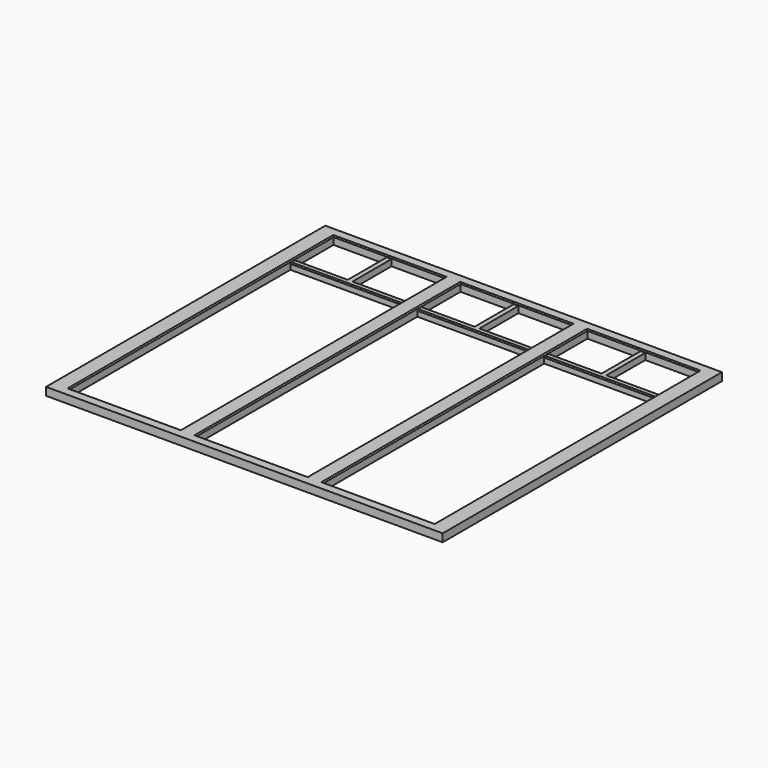
from build123d import *

# Parameters (mm, degrees)
F0_W      = 2500
F0_H      = 2200
F1_DEPTH  = 50
F0_W_2    = 30
F0_H_2    = 300
F2_DEPTH  = 40
F3_SIZE   = 7
F3_2_SIZE = 7
F3_3_SIZE = 7
F3_4_SIZE = 7


# Not quite as in the source:
# - a feature names something its author has since deleted; it is built from what else it names


with BuildPart() as f1:
    # F0 (on Top) → F1 (new body)
    with BuildSketch(Plane.XY):
        with Locations((321.0913794215, -344.7952681527)):
            Rectangle(F0_W, F0_H)
        Polygon((-828.9086205785, 395.2047318473), (-828.9086205785, 695.2047318473), (-493.9086205785, 695.2047318473), (-463.9086205785, 695.2047318473), (-128.9086205785, 695.2047318473), (-28.9086205785, 695.2047318473), (306.0913794215, 695.2047318473), (336.0913794215, 695.2047318473), (671.0913794215, 695.2047318473), (771.0913794215, 695.2047318473), (1106.0913794215, 695.2047318473), (1136.0913794215, 695.2047318473), (1471.0913794215, 695.2047318473), (1471.0913794215, 395.2047318473), (1471.0913794215, 355.2047318473), (1471.0913794215, -1384.7952681527), (771.0913794215, -1384.7952681527), (671.0913794215, -1384.7952681527), (-28.9086205785, -1384.7952681527), (-128.9086205785, -1384.7952681527), (-828.9086205785, -1384.7952681527), (-828.9086205785, 355.2047318473), align=None, mode=Mode.SUBTRACT)
        Polygon((-28.9086205785, 695.2047318473), (-128.9086205785, 695.2047318473), (-128.9086205785, 395.2047318473), (-128.9086205785, 355.2047318473), (-128.9086205785, -1384.7952681527), (-28.9086205785, -1384.7952681527), (-28.9086205785, 355.2047318473), (-28.9086205785, 395.2047318473), align=None)
        Polygon((671.0913794215, 355.2047318473), (671.0913794215, -1384.7952681527), (771.0913794215, -1384.7952681527), (771.0913794215, 355.2047318473), (771.0913794215, 395.2047318473), (771.0913794215, 695.2047318473), (671.0913794215, 695.2047318473), (671.0913794215, 395.2047318473), align=None)
    extrude(amount=F1_DEPTH)

    # F3
    f3_edges = [f1.edges().sort_by_distance(p)[0] for p in [
        (-828.908621, -344.795268, 50),
        (-478.908621, 695.204732, 50),
        (-128.908621, -344.795268, 50),
        (-28.908621, -344.795268, 50),
        (321.091379, 695.204732, 50),
        (771.091379, -344.795268, 50),
        (1121.091379, 695.204732, 50),
        (671.091379, -344.795268, 50),
        (1471.091379, -344.795268, 50),
        (321.091379, -1384.795268, 50),
        (1121.091379, -1384.795268, 50),
        (-478.908621, -1384.795268, 50),
    ]]
    chamfer(f3_edges, length=F3_SIZE)


with BuildPart() as f2:
    # F0 (on Top) → F2 (new body)
    with BuildSketch(Plane.XY):
        Polygon((-493.9086205785, 395.2047318473), (-828.9086205785, 395.2047318473), (-828.9086205785, 355.2047318473), (-128.9086205785, 355.2047318473), (-128.9086205785, 395.2047318473), (-463.9086205785, 395.2047318473), align=None)
        with Locations((-478.9086205785, 545.2047318473)):
            Rectangle(F0_W_2, F0_H_2)
    extrude(amount=F2_DEPTH)

    # F3#2
    f3_2_edges = [f2.edges().sort_by_distance(p)[0] for p in [
        (-478.908621, 355.204732, 40),
        (-661.408621, 395.204732, 40),
        (-296.408621, 395.204732, 40),
    ]]
    chamfer(f3_2_edges, length=F3_2_SIZE)


with BuildPart() as f2b:
    # F0 (on Top) → F2, piece 2 (new body)
    with BuildSketch(Plane.XY):
        Polygon((306.0913794215, 395.2047318473), (-28.9086205785, 395.2047318473), (-28.9086205785, 355.2047318473), (671.0913794215, 355.2047318473), (671.0913794215, 395.2047318473), (336.0913794215, 395.2047318473), align=None)
        with Locations((321.0913794215, 545.2047318473)):
            Rectangle(F0_W_2, F0_H_2)
    extrude(amount=F2_DEPTH)

    # F3#3
    f3_3_edges = [f2b.edges().sort_by_distance(p)[0] for p in [
        (321.091379, 355.204732, 40),
        (138.591379, 395.204732, 40),
        (503.591379, 395.204732, 40),
    ]]
    chamfer(f3_3_edges, length=F3_3_SIZE)


with BuildPart() as f2c:
    # F0 (on Top) → F2, piece 3 (new body)
    with BuildSketch(Plane.XY):
        Polygon((771.0913794215, 395.2047318473), (771.0913794215, 355.2047318473), (1471.0913794215, 355.2047318473), (1471.0913794215, 395.2047318473), (1136.0913794215, 395.2047318473), (1106.0913794215, 395.2047318473), align=None)
        with Locations((1121.0913794215, 545.2047318473)):
            Rectangle(F0_W_2, F0_H_2)
    extrude(amount=F2_DEPTH)

    # F3#4
    f3_4_edges = [f2c.edges().sort_by_distance(p)[0] for p in [
        (1303.591379, 395.204732, 40),
        (938.591379, 395.204732, 40),
        (1121.091379, 355.204732, 40),
    ]]
    chamfer(f3_4_edges, length=F3_4_SIZE)


solid = Compound([f1.part, f2.part, f2b.part, f2c.part])
